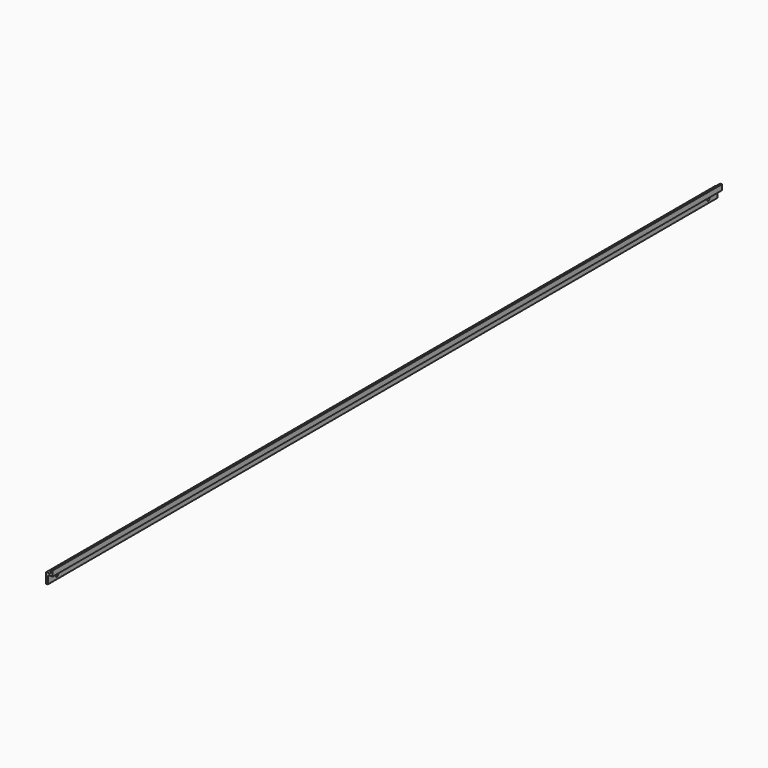
from build123d import *

# Parameters (mm, degrees)
F0_W     = 8.89
F0_H     = 18.7198
F1_DEPTH = 1143
F2_W     = 6.35
F2_H     = 4.7498
F2_H_2   = 11.43
F3_DEPTH = 1143.001
F4_R     = 0.127
F6_DEPTH = 1143.001
F7_R     = 2.032
F8_DEPTH = 2.54


# Not quite as in the source:
# - a pattern or mirror of a feature is missing from the dataset's text; its kind, count and spacing are read off the source's solid


with BuildPart() as f1:
    # F0 (on Front) → F1 (new body)
    with BuildSketch(Plane.XZ):
        with Locations((4.445, 9.3599)):
            Rectangle(F0_W, F0_H)
    extrude(amount=F1_DEPTH)

    # F2 (on face) → F3 (cut, through all)
    with BuildSketch(Plane.XZ.offset(1143)):
        with Locations((3.175, 16.3449)):
            Rectangle(F2_W, F2_H)
        with Locations((5.715, 5.715)):
            Rectangle(F2_W, F2_H_2)
    extrude(amount=-F3_DEPTH, mode=Mode.SUBTRACT)

    # F4
    f4_edges = [f1.edges().sort_by_distance(p)[0] for p in [
        (6.35, -571.5, 18.7198),
        (8.89, -571.5, 18.7198),
        (2.54, -571.5, 0),
        (0, -571.5, 0),
        (0, -571.5, 13.97),
    ]]
    fillet(f4_edges, radius=F4_R)

    # F7 (on face) → F8 (cut, through all)
    with BuildSketch(Plane.YZ.offset(2.54)):
        with Locations((-1127.76, 5.08)):
            Circle(F7_R)
        with Locations((-15.24, 5.08)):
            Circle(F7_R)
    extrude(amount=-F8_DEPTH, mode=Mode.SUBTRACT)


with BuildPart() as f6:
    # F5 (on face) → F6 (new body, through all)
    with BuildSketch(Plane.XZ.offset(1143)):
        Polygon((2.54, 10.16), (3.81, 11.43), (2.54, 11.43), align=None)
    extrude(amount=-F6_DEPTH)

    # F6_copies: F6 across plane


with BuildPart() as f6_1:
    add(f6.part)
    add(f6.part.mirror(Plane.ZX.offset(-571.401074)))


solid = Compound([f1.part, f6_1.part])
